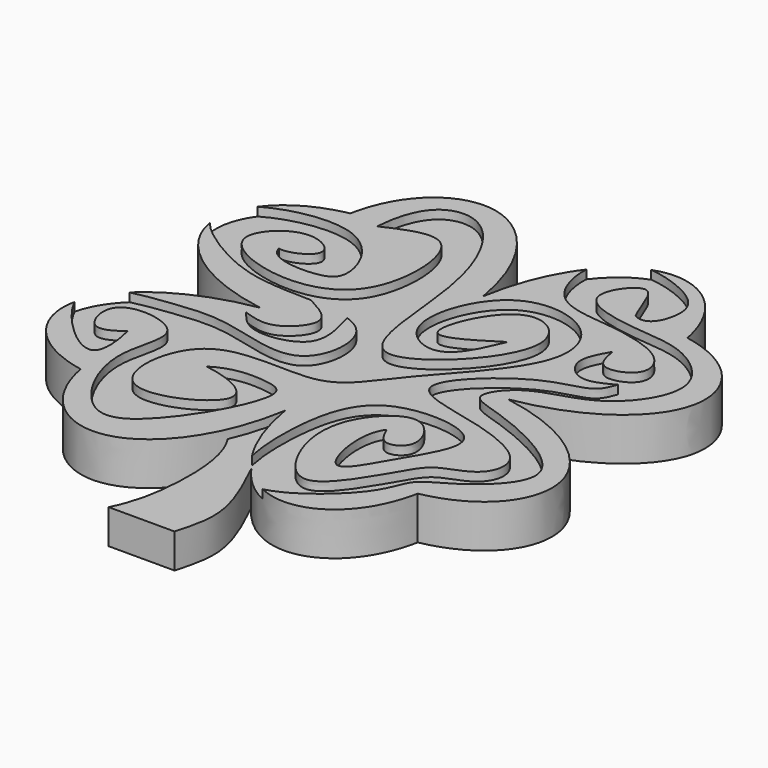
from build123d import *

# Parameters (mm, degrees)
F1_DEPTH = 12.7
F4_COUNT = 4
F4_ANGLE = 270
F6_DEPTH = 10.16
F8_DEPTH = 2.54


# Not quite as in the source:
# - the dataset's text gives a spline's control points without its knots; the knots are read off the source's solid


with BuildPart() as f1:
    # F0 (on Top) → F1 (new body)
    with BuildSketch(Plane.XY):
        with BuildLine():
            add(Edge.make_bspline(
                [(-36.5691743791, 0), (-57.5325042009, 3.4879909363), (-82.2126755416, 24.2816366213), (-65.4620230198, 46.6733649373), (-49.7792437673, 49.7792437673)],
                knots=[0, 0, 0, 0, 0.5390938735, 1, 1, 1, 1], degree=3))
            Line((-36.5691743791, 0), (0, 0))
            Line((0, 0), (-49.7792437673, 49.7792437673))
        make_face()
    extrude(amount=F1_DEPTH)

    # F2: F1 across face


with BuildPart() as f1_1:
    add(f1.part)
    add(f1.part.mirror(Plane(origin=(-24.8896218836, 24.8896218836, 6.35), x_dir=(-0.7071067812, 0.7071067812, 0), z_dir=(0.7071067812, 0.7071067812, 0))))

    # F4: F1 ×4 about axis
    f4_axis = Axis((0, 0, 17.2648541629), (0, 0, 1))


with BuildPart() as f1_2:
    add(f1_1.part)
    for i in range(1, F4_COUNT):
        add(f1_1.part.rotate(f4_axis, i * F4_ANGLE / (F4_COUNT - 1)))

    # F5 (on Top) → F6 (join)
    with BuildSketch(Plane.XY):
        with BuildLine():
            add(Edge.make_bspline(
                [(0, -36.5691743791), (1.5994040624, -46.1818240362), (4.8224141221, -54.1841848757), (8.9693114745, -60.1537320031)],
                knots=[0, 0, 0, 0, 0.2471993039, 0.2471993039, 0.2471993039, 0.2471993039], degree=3))
            add(Edge.make_bspline(
                [(0, -36.5691743791), (-0.9598021929, -42.3377243267), (-2.5042971683, -47.5263772726), (-4.4822701915, -52.0438222523)],
                knots=[0, 0, 0, 0, 0.1483442737, 0.1483442737, 0.1483442737, 0.1483442737], degree=3))
            add(Edge.make_bspline(
                [(-4.4822701915, -52.0438222523), (-0.3657960993, -58.4274790843), (0.8663677136, -75.0833095194), (-1.3361890327, -88.9867105998), (-4.6823425218, -95.7678183913)],
                knots=[0, 0, 0, 0, 0.5077116323, 1, 1, 1, 1], degree=3))
            Line((-4.6823425218, -95.7678183913), (14.7543838248, -95.7678183913))
            add(Edge.make_bspline(
                [(8.9693114745, -60.1537320031), (12.5335313957, -67.6040906429), (18.9500764, -80.9656287943), (16.0405576708, -91.2250874302), (14.7543838248, -95.7678183913)],
                knots=[0, 0, 0, 0, 0.5571227043, 1, 1, 1, 1], degree=3))
        make_face()
    extrude(amount=F6_DEPTH)

    # F7 (on face) → F8 (cut)
    with BuildSketch(Plane.XY.offset(12.7)):
        with BuildLine():
            add(Edge.make_bspline(
                [(-40.9096889198, 48.5747121274), (-40.4980060973, 54.4612315191), (-37.6593086249, 65.3470099902), (-21.4745890193, 67.8541178952), (-5.4591771434, 39.7950732001), (-8.441950326, -17.0461155053), (35.2130466512, 25.6909951941), (10.8569238229, 42.9467529137), (-3.478718201, 8.2126534489), (11.4809961233, 17.754333856), (18.7105406076, 22.3229814791)],
                knots=[0, 0, 0, 0, 0.1059622614, 0.1941390807, 0.3438088633, 0.50716741, 0.6645014534, 0.7675402942, 0.8906043724, 1, 1, 1, 1], degree=3))
            add(Edge.make_bspline(
                [(-51.6652688384, 25.777855888), (-48.4352505, 25.2451919112), (-38.1602504989, 30.2089280661), (-52.0203730291, 38.916077621), (-66.6802847112, 24.5772026744), (-47.4712345486, 13.1362518804), (-17.7286252383, 16.3228225718), (-19.2985278154, 58.7087749334), (-35.0107539886, 51.3187872243), (-40.9096889198, 48.5747121274)],
                knots=[0, 0, 0, 0, 0.1105388033, 0.2190546311, 0.3497734037, 0.4922968496, 0.668587798, 0.8551375666, 1, 1, 1, 1], degree=3))
            add(Edge.make_bspline(
                [(-29.7772348165, 10.2924870865), (-32.4263115499, 10.4016118636), (-43.9871416548, 10.5371550805), (-57.0922695913, 13.2107968725), (-87.3272579837, 34.9461191438), (-40.1874399837, 51.0698272915), (-28.9894496144, 24.7812529377), (-36.3237815611, 20.0714672558), (-50.6689773411, 21.0467340984), (-51.6652688384, 25.777855888)],
                knots=[0.5424249266, 0.5424249266, 0.5424249266, 0.5424249266, 0.5653534026, 0.6430999082, 0.7225663475, 0.8161633484, 0.8918762745, 0.9352201018, 1, 1, 1, 1], degree=3))
            add(Edge.make_bspline(
                [(-17.7366641926, 8.5464966924), (-21.2300566221, 9.7404250869), (-25.524427018, 10.1172989929), (-29.7772348165, 10.2924870865)],
                knots=[0.5056157242, 0.5056157242, 0.5056157242, 0.5056157242, 0.5424249266, 0.5424249266, 0.5424249266, 0.5424249266], degree=3))
            add(Edge.make_bspline(
                [(-53.156144917, -28.1502474099), (-52.0267455305, -32.3092497522), (-50.2989245665, -45.570049298), (-66.3950956482, -34.3142195553), (-79.136602485, -14.3471554495), (-52.8080746506, -10.803908412), (-37.8837532136, -9.1795733173), (-10.4854321398, -19.9036464958), (-7.7945773019, 3.2511421308), (-15.3695875491, 7.7375065564), (-17.7366641926, 8.5464966924)],
                knots=[0, 0, 0, 0, 0.0580253435, 0.1189641715, 0.1895111401, 0.2616253839, 0.3322257147, 0.4111182033, 0.480674294, 0.5056157242, 0.5056157242, 0.5056157242, 0.5056157242], degree=3))
            add(Edge.make_bspline(
                [(-27.9155354947, -30.6582842022), (-22.6364423701, -27.2146564615), (-13.3061244116, -27.2897813724), (-2.0432780007, -30.3615498026), (-24.5091615606, -69.3174761805), (-40.9083450045, -60.2730965577), (-50.3248853139, -38.7830509465), (-41.2166408779, -21.4528597178), (-57.4087309955, -16.9508514159), (-65.3876349105, -21.412507814), (-61.460287185, -33.4748209423), (-55.6843257393, -30.1574213288), (-53.156144917, -28.1502474099)],
                knots=[0, 0, 0, 0, 0.1070959153, 0.1772451541, 0.3406794689, 0.4395595908, 0.5683390444, 0.674726271, 0.769997047, 0.8442794976, 0.9239381342, 1, 1, 1, 1], degree=3))
            add(Edge.make_bspline(
                [(18.7105406076, 22.3229814791), (16.0730638131, 16.1961767952), (11.1477724767, 4.5761357599), (-7.7892575026, 14.4092609843), (3.2193113207, 45.0935443433), (29.7874315566, 41.1949800019), (36.6627196166, 19.8561016549), (9.7064590159, -5.7243694188), (-0.6341466405, -24.926857558), (-39.4176086089, -14.2240691765), (-43.027838287, -57.9621250683), (-3.8172273743, -39.1993092809), (-20.0044060123, -31.7989823887), (-27.9155354947, -30.6582842022)],
                knots=[0, 0, 0, 0, 0.079841203, 0.1508770503, 0.2491784087, 0.3380523515, 0.4186939964, 0.5349017295, 0.6227133417, 0.7312277254, 0.8260020459, 0.9201541725, 1, 1, 1, 1], degree=3))
        make_face()
        with BuildLine():
            add(Edge.make_bspline(
                [(-17.7366641926, 8.5464966924), (-21.2300566221, 9.7404250869), (-25.524427018, 10.1172989929), (-29.7772348165, 10.2924870865)],
                knots=[0.5056157242, 0.5056157242, 0.5056157242, 0.5056157242, 0.5424249266, 0.5424249266, 0.5424249266, 0.5424249266], degree=3))
            add(Edge.make_bspline(
                [(-29.7772348165, 10.2924870865), (-25.9300253771, 8.228077581), (-18.294367339, 4.1577524525), (-28.3287224415, -6.9666952947), (-34.6228401519, -4.8265293787), (-37.7005189657, -3.7812164519)],
                knots=[0, 0, 0, 0, 0.3420245332, 0.6784264033, 1, 1, 1, 1], degree=3))
            add(Edge.make_bspline(
                [(-37.7005189657, -3.7812164519), (-35.8868211778, -6.1438763128), (-31.8251797554, -11.4424939071), (-12.9101200438, -8.1622076485), (-16.1232748224, 2.9093751488), (-17.7366641926, 8.5464966924)],
                knots=[0, 0, 0, 0, 0.2841362427, 0.6376842332, 1, 1, 1, 1], degree=3))
        make_face()
        with BuildLine():
            add(Edge.make_bspline(
                [(51.8795251846, 21.5093474835), (51.1849059507, 19.6542638933), (49.3679880711, 14.8022474206), (35.3496137735, 14.4344673908), (9.4661054928, -9.0620369377), (37.6153490939, -13.040675314), (58.6973129225, -21.0984684577), (55.8240483078, -33.3793056135), (44.9882466531, -36.1325545311), (40.5876589607, -40.9765140294), (26.9106216553, -67.9697615844), (13.0313080169, -49.4945411785), (11.7013487965, -30.3642704699), (27.4833962168, -16.1850289186), (36.4242531555, -31.6081535208), (27.4302471579, -36.2486349111), (25.3164505169, -31.6652648808), (24.2704767734, -29.3995719403)],
                knots=[0, 0, 0, 0, 0.044305533, 0.1132718869, 0.2043586403, 0.2852790957, 0.3711805332, 0.4246257417, 0.4820866513, 0.5327473446, 0.6216252951, 0.6923355316, 0.7740137657, 0.8456320872, 0.9078234653, 0.9533047321, 1, 1, 1, 1], degree=3))
            add(Edge.make_bspline(
                [(24.2704767734, -29.3995719403), (20.2099885722, -34.3177653523), (24.8591316935, -58.936675051), (34.8231424698, -38.9165563203), (48.9448610394, -18.2370354479), (14.6416920474, -15.0609054046), (4.739747421, -36.7114357891), (9.0845093727, -83.5953613522), (43.041970037, -56.5063427884), (43.96650526, -45.0639837911), (54.0264254563, -41.2767946907), (75.3415988208, -22.6542644149), (40.9700071317, -6.5127629747), (27.5549127809, -4.2144499187), (36.6059850221, 8.5570058863), (55.2038244516, 9.6471847737), (69.6744543409, 30.8922598853), (52.7696703843, 45.7323490484), (37.5371976794, 45.3283425672), (14.9813638777, 50.170378809), (28.7825505229, 68.931163682), (31.1798641145, 55.3854357122), (33.5494093597, 50.9009547532)],
                knots=[0, 0, 0, 0, 0.0539735614, 0.0972532003, 0.1495063667, 0.2051890968, 0.2621562558, 0.3298191866, 0.3937358436, 0.4328600297, 0.4708177921, 0.5229687899, 0.5883425316, 0.6271097555, 0.6648908776, 0.7164265147, 0.7697882696, 0.8189931284, 0.8682516446, 0.9169120273, 0.9565168928, 1, 1, 1, 1], degree=3))
            add(Edge.make_bspline(
                [(33.5494093597, 50.9009547532), (38.0502827466, 48.4326928854), (42.6402538599, 58.4982343074), (37.2020157325, 68.2576016849), (7.4410769132, 76.1358959348), (10.7860865225, 43.9943131205), (32.0937332413, 44.1520664133), (51.2812592828, 39.3926048908), (54.0389700872, 28.4834507833), (42.1880157815, 24.4120878949), (41.1187631264, 30.8304031475), (40.6531281769, 33.6338542402)],
                knots=[0, 0, 0, 0, 0.0938448237, 0.1952845619, 0.3392827768, 0.4753737734, 0.6098093387, 0.7430951369, 0.827504385, 0.9159419446, 1, 1, 1, 1], degree=3))
            add(Edge.make_bspline(
                [(40.6531281769, 33.6338542402), (38.8973861837, 30.5838567266), (35.5443557637, 24.7591202429), (43.0313209062, 16.8628983603), (48.852759776, 19.9199050344), (51.8795251846, 21.5093474835)],
                knots=[0, 0, 0, 0, 0.345416529, 0.6596596389, 1, 1, 1, 1], degree=3))
        make_face()
    extrude(amount=-F8_DEPTH, mode=Mode.SUBTRACT)


solid = f1_2.part
